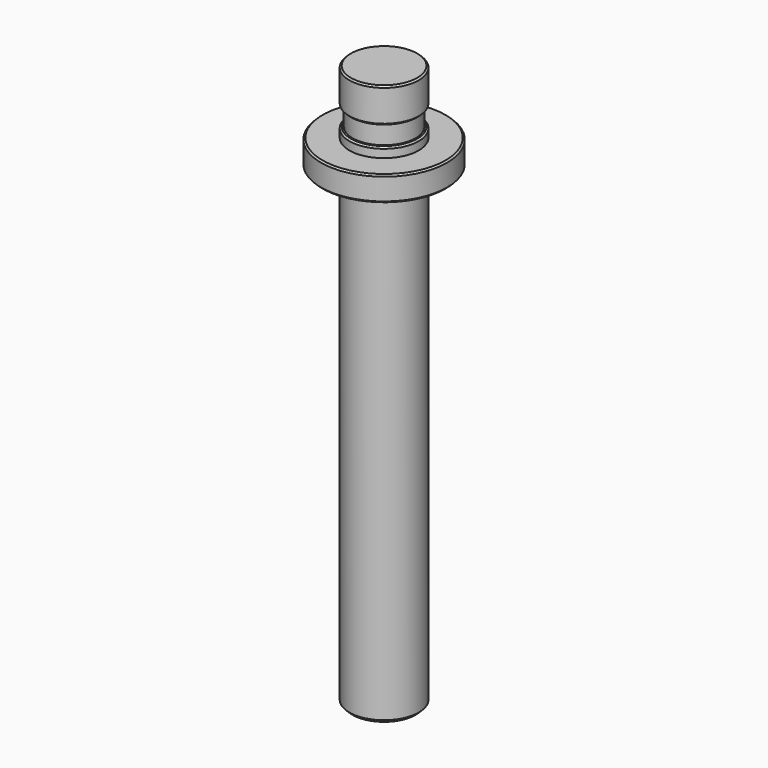
from build123d import *

# Parameters (mm, degrees)
F0_R      = 11
F1_DEPTH  = 150
F2_R      = 20
F3_DEPTH  = 7.9
F4_R      = 11
F5_DEPTH  = 3.1
F6_R      = 10
F7_DEPTH  = 6
F8_R      = 11
F9_DEPTH  = 11
F11_D     = 10.3
F11_DEPTH = 35
F11_TIP   = 3.094432188
F12_SIZE  = 1
F13_SIZE  = 0.5


with BuildPart() as f1:
    # F0 (on Top) → F1 (new body)
    with BuildSketch(Plane.XY):
        Circle(F0_R)
    extrude(amount=F1_DEPTH)

    # F2 (on face) → F3 (join)
    with BuildSketch(Plane.XY.offset(150)):
        Circle(F2_R)
    extrude(amount=F3_DEPTH)

    # F4 (on face) → F5 (join)
    with BuildSketch(Plane.XY.offset(157.9)):
        Circle(F4_R)
    extrude(amount=F5_DEPTH)

    # F6 (on face) → F7 (join)
    with BuildSketch(Plane.XY.offset(161)):
        Circle(F6_R)
    extrude(amount=F7_DEPTH)

    # F8 (on face) → F9 (join)
    with BuildSketch(Plane.XY.offset(167)):
        Circle(F8_R)
    extrude(amount=F9_DEPTH)

    # F11
    with Locations(Plane(origin=(0, 0, 0), x_dir=(1, 0, 0), z_dir=(0, 0, -1))):
        with Locations((0, 0)):
            Hole(F11_D / 2, depth=F11_DEPTH)
            with Locations((0, 0, -(F11_DEPTH + F11_TIP / 2))):  # 118° drill point
                Cone(0, F11_D / 2, F11_TIP, mode=Mode.SUBTRACT)

    # F12
    f12_edges = [f1.edges().sort_by_distance(p)[0] for p in [
        (-11, 0, 0),
        (-5.15, 0, 0),
    ]]
    chamfer(f12_edges, length=F12_SIZE)

    # F13
    f13_edges = [f1.edges().sort_by_distance(p)[0] for p in [
        (-20, 0, 150),
        (-20, 0, 157.9),
        (-11, 0, 161),
        (-11, 0, 167),
        (-11, 0, 178),
    ]]
    chamfer(f13_edges, length=F13_SIZE)


solid = f1.part
